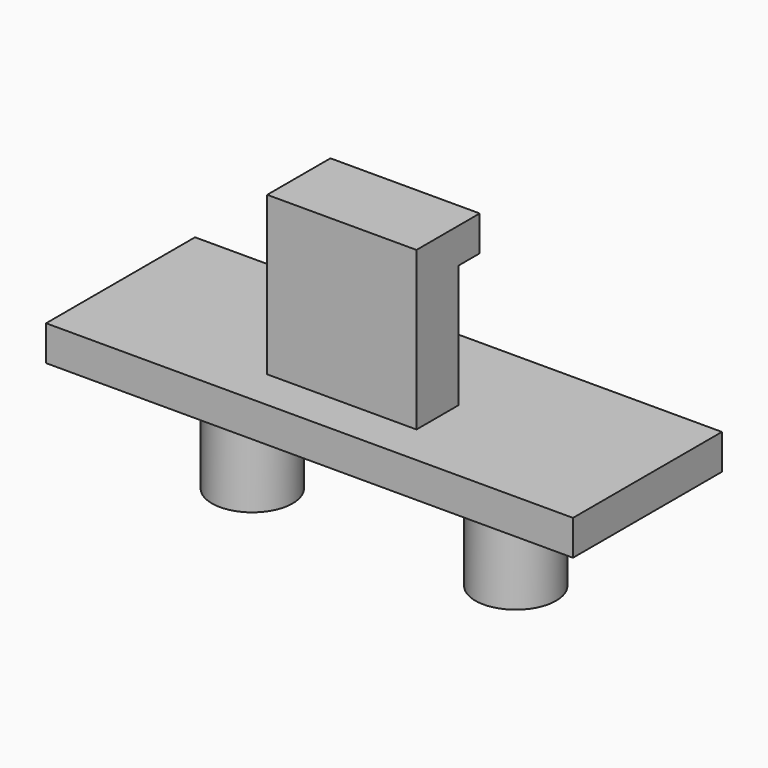
from build123d import *

# Parameters (mm, degrees)
F0_W     = 15
F0_H     = 10.6
F0_R     = 2.3
F1_DEPTH = 2
F2_DEPTH = 8
F3_W     = 8.5
F3_H     = 3
F4_DEPTH = 9
F5_START = 7
F3_H_2   = 1.5
F5_DEPTH = 2


# Not quite as in the source:
# - a feature names something its author has since deleted; it is built from what else it names


with BuildPart() as f1:
    # F0 (on Top) → F1 (new body)
    with BuildSketch(Plane.XY):
        with Locations((-7.5, 0)):
            Rectangle(F0_W, F0_H)
        with Locations((-7.5, 0)):
            Circle(F0_R, mode=Mode.SUBTRACT)
        with Locations((7.5, 0)):
            Rectangle(F0_W, F0_H)
        with Locations((7.5, 0)):
            Circle(F0_R, mode=Mode.SUBTRACT)
    extrude(amount=-F1_DEPTH)

    # F0 (on Top) → F2 (join)
    with BuildSketch(Plane.XY):
        with Locations((-7.5, 0)):
            Circle(F0_R)
        with Locations((7.5, 0)):
            Circle(F0_R)
    extrude(amount=-F2_DEPTH)

    # F3 (on Top) → F4 (join)
    with BuildSketch(Plane.XY):
        with Locations((0, -1.5)):
            Rectangle(F3_W, F3_H)
    extrude(amount=F4_DEPTH)

    # F3 (on Top) → F5 (join)
    with BuildSketch(Plane.XY.offset(F5_START)):
        with Locations((0, 0.75)):
            Rectangle(F3_W, F3_H_2)
    extrude(amount=F5_DEPTH)


solid = f1.part
